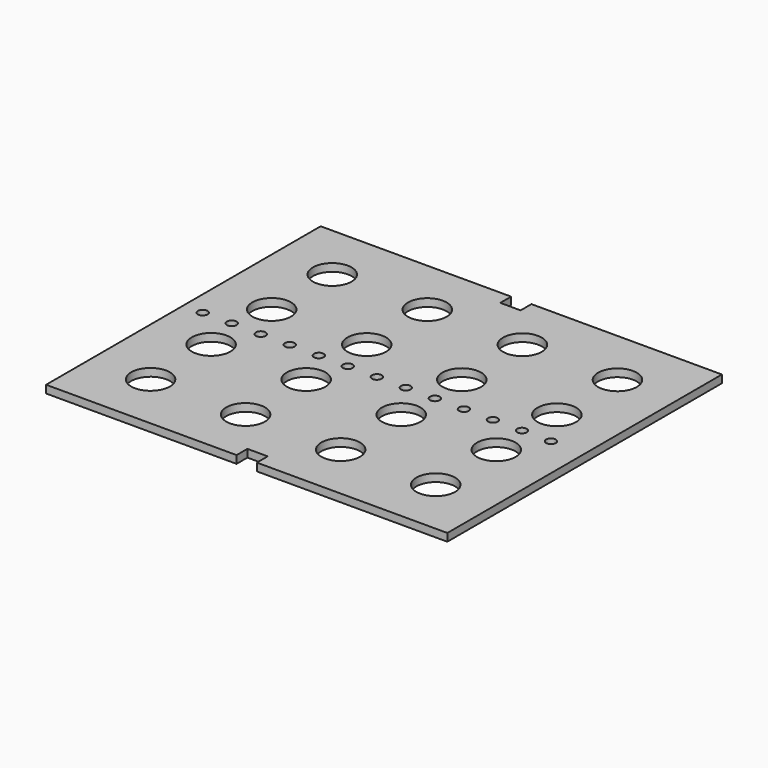
from build123d import *

# Parameters (mm, degrees)
F0_R     = 10
F1_DEPTH = 4
F2_D     = 5


# Not quite as in the source:
# - a feature names something its author has since deleted; it is built from what else it names
# - the program builds the solid bodies; features that only make, move or delete a surface that nothing else refers to are left out


with BuildPart() as f1:
    # F0 (on Top) → F1 (new body)
    with BuildSketch(Plane.XY):
        Polygon((1.9552472353, 143.8201326668), (-96.4947527647, 143.8201326668), (-96.4947527647, -33.5798673332), (1.9552472353, -33.5798673332), (1.9552472353, -26.5798673332), (12.4552472353, -26.5798673332), (12.4552472353, -33.5798673332), (110.9052472353, -33.5798673332), (110.9052472353, 143.8201326668), (12.4552472353, 143.8201326668), (12.4552472353, 136.8201326668), (1.9552472353, 136.8201326668), align=None)
        with Locations((-66.4946527647, -3.5798663332)):
            Circle(F0_R, mode=Mode.SUBTRACT)
        with Locations((-17.3613527647, -3.5798663332)):
            Circle(F0_R, mode=Mode.SUBTRACT)
        with Locations((-66.4946527647, 35.5534666668)):
            Circle(F0_R, mode=Mode.SUBTRACT)
        with Locations((-17.3613527647, 35.5534666668)):
            Circle(F0_R, mode=Mode.SUBTRACT)
        with Locations((31.7719472353, -3.5798663332)):
            Circle(F0_R, mode=Mode.SUBTRACT)
        with Locations((80.9052472353, -3.5798663332)):
            Circle(F0_R, mode=Mode.SUBTRACT)
        with Locations((31.7719472353, 35.5534666668)):
            Circle(F0_R, mode=Mode.SUBTRACT)
        with Locations((80.9052472353, 35.5534666668)):
            Circle(F0_R, mode=Mode.SUBTRACT)
        with Locations((-66.4946527647, 74.6867996668)):
            Circle(F0_R, mode=Mode.SUBTRACT)
        with Locations((-17.3613527647, 74.6867996668)):
            Circle(F0_R, mode=Mode.SUBTRACT)
        with Locations((-66.4946527647, 113.8201326668)):
            Circle(F0_R, mode=Mode.SUBTRACT)
        with Locations((-17.3613527647, 113.8201326668)):
            Circle(F0_R, mode=Mode.SUBTRACT)
        with Locations((31.7719472353, 74.6867996668)):
            Circle(F0_R, mode=Mode.SUBTRACT)
        with Locations((80.9052472353, 74.6867996668)):
            Circle(F0_R, mode=Mode.SUBTRACT)
        with Locations((31.7719472353, 113.8201326668)):
            Circle(F0_R, mode=Mode.SUBTRACT)
        with Locations((80.9052472353, 113.8201326668)):
            Circle(F0_R, mode=Mode.SUBTRACT)
    extrude(amount=F1_DEPTH)

    # F2 (through all)
    with Locations(Plane(origin=(0, 0, 0), x_dir=(1, 0, 0), z_dir=(0, 0, -1))):
        with Locations((18.5052472353, -55.1201326668), (-11.4947527647, -55.1201326668), (-56.4947527647, -55.1201326668), (93.5052472353, -55.1201326668), (-26.4947527647, -55.1201326668), (78.5052472353, -55.1201326668), (63.5052472353, -55.1201326668), (-71.4947527647, -55.1201326668), (33.5052472353, -55.1201326668), (-41.4947527647, -55.1201326668), (3.5052472353, -55.1201326668), (48.5052472353, -55.1201326668), (-86.4947527647, -55.1201326668)):
            Hole(F2_D / 2)


solid = f1.part
